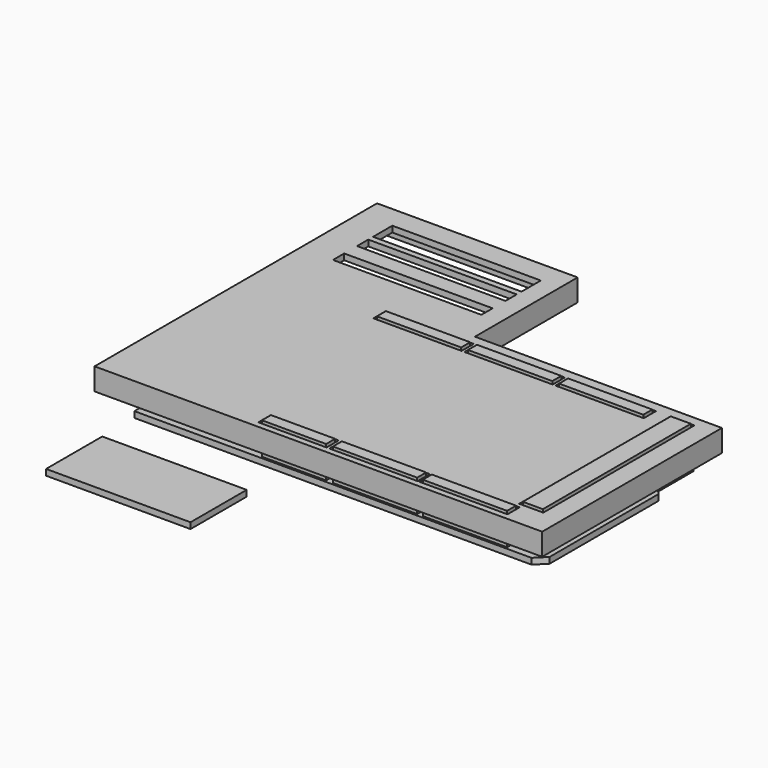
from build123d import *

# Parameters (mm, degrees)
F1_DEPTH  = 1.5
F2_SIZE   = 2.49999
F3_W      = 21
F3_H      = 2.8
F3_W_2    = 5
F3_H_2    = 46.1
F3_W_3    = 16
F4_DEPTH  = 8
F5_W      = 36
F5_H      = 17.5
F6_DEPTH  = 1.5
F9_W      = 17
F9_H      = 3.8
F9_W_2    = 22
F9_W_3    = 37
F9_H_2    = 3.5
F9_W_4    = 6
F9_H_3    = 47.1
F10_DEPTH = 1.5
F12_DEPTH = 4


# Not quite as in the source:
# - a fillet or chamfer is up to 0.001 mm smaller than in the source, because OpenCascade refuses the exact size
# - a feature names something its author has since deleted; it is built from what else it names


with BuildPart() as f1:
    # F0 (on Top) → F1 (new body)
    with BuildSketch(Plane.XY):
        Polygon((51.935759174, 26.5), (-47.064240826, 26.5), (-47.064240826, -26.5), (54.435759174, -26.5), (54.435759174, 12.5), (51.935759174, 12.5), align=None)
    extrude(amount=F1_DEPTH)

    # F2 (size 2.5 in the source; OpenCascade refuses exactly that, so slightly less here)
    f2_edges = [f1.edges().sort_by_distance(p)[0] for p in [
        (54.435759, 12.5, 0.75),
        (51.935759, 26.5, 0.75),
        (54.435759, -26.5, 0.75),
    ]]
    chamfer(f2_edges, length=F2_SIZE)

    # F3 (on face) → F4 (join)
    with BuildSketch(Plane.XY.offset(1.5)):
        with Locations((-15.064240826, 23.6)):
            Rectangle(F3_W, F3_H)
        with Locations((7.635759174, 23.6)):
            Rectangle(F3_W, F3_H)
        with Locations((30.335759174, 23.6)):
            Rectangle(F3_W, F3_H)
        with Locations((47.935759174, 1.95)):
            Rectangle(F3_W_2, F3_H_2)
        with Locations((34.935759174, -24.6)):
            Rectangle(F3_W, F3_H)
        with Locations((12.535759174, -24.6)):
            Rectangle(F3_W, F3_H)
        with Locations((-7.664240826, -24.6)):
            Rectangle(F3_W_3, F3_H)
    extrude(amount=F4_DEPTH)


with BuildPart() as f6:
    # F5 (on Top) → F6 (new body)
    with BuildSketch(Plane.XY):
        with Locations((-29.064240826, -45.25)):
            Rectangle(F5_W, F5_H)
    extrude(amount=-F6_DEPTH)


with BuildPart() as f10:
    # F9 (on offset) → F10 (new body)
    with BuildSketch(Plane.XY.offset(7.6)):
        Polygon((-55.7806417346, 28), (-55.7806417346, -28), (-5.7806417346, -28), (55.7806417346, -28), (55.7806417346, 28), (-5.7806417346, 28), (-5.7806417346, 60), (-55.7806417346, 60), align=None)
        with Locations((-7.664240826, -24.6)):
            Rectangle(F9_W, F9_H, mode=Mode.SUBTRACT)
        with Locations((12.535759174, -24.6)):
            Rectangle(F9_W_2, F9_H, mode=Mode.SUBTRACT)
        with Locations((34.935759174, -24.6)):
            Rectangle(F9_W_2, F9_H, mode=Mode.SUBTRACT)
        with Locations((-15.064240826, 23.6)):
            Rectangle(F9_W_2, F9_H, mode=Mode.SUBTRACT)
        with Locations((-29.064240826, 37.75)):
            Rectangle(F9_W_3, F9_H_2, mode=Mode.SUBTRACT)
        with Locations((-29.064240826, 45.25)):
            Rectangle(F9_W_3, F9_H_2, mode=Mode.SUBTRACT)
        Polygon((-47.564240826, 48.5), (-47.564240826, 51.5), (-47.564240826, 54.5), (-10.564240826, 54.5), (-10.564240826, 51.5), (-10.564240826, 48.5), align=None, mode=Mode.SUBTRACT)
        with Locations((7.635759174, 23.6)):
            Rectangle(F9_W_2, F9_H, mode=Mode.SUBTRACT)
        with Locations((47.935759174, 1.95)):
            Rectangle(F9_W_4, F9_H_3, mode=Mode.SUBTRACT)
        with Locations((30.335759174, 23.6)):
            Rectangle(F9_W_2, F9_H, mode=Mode.SUBTRACT)
    extrude(amount=F10_DEPTH)

    # F11 (on face) → F12 (join)
    with BuildSketch(Plane(origin=(0, 0, 7.6), x_dir=(1, 0, 0), z_dir=(0, 0, -1))):
        Polygon((-55.7806417346, 28), (-55.7806417346, -28), (-55.7806417346, -60), (-5.7806417346, -60), (-5.7806417346, -28), (55.7806417346, -28), (55.7806417346, 28), (-5.7806417346, 28), align=None)
        Polygon((-54.5806417346, -58.8), (-54.5806417346, -30), (-54.5806417346, 26.8), (-6, 26.8), (54.5806417346, 26.8), (54.5806417346, -26.8), (-6.9806417346, -26.8), (-6.9806417346, -58.8), align=None, mode=Mode.SUBTRACT)
    extrude(amount=F12_DEPTH)


solid = Compound([f1.part, f6.part, f10.part])
